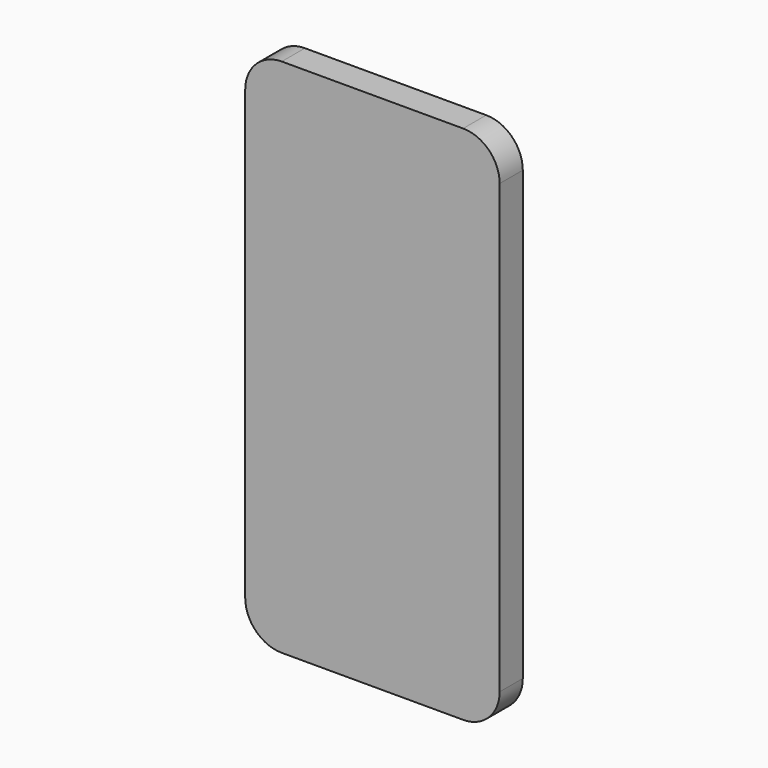
from build123d import *

# Parameters (mm, degrees)
F0_W         = 69.6
F0_H         = 142.4
F1_DEPTH     = 7.9
F2_R         = 10
F3_TEXT_SIZE = 14.5033047895
F4_DEPTH     = 0.5


# Not quite as in the source:
# - Text() gives the source's letters only with a copy of the font that has no kerning and outlines rounded to 1/6400 em; it was checked with that copy


with BuildPart() as f1:
    # F0 (on Front) → F1 (new body)
    with BuildSketch(Plane.XZ):
        Rectangle(F0_W, F0_H)
    extrude(amount=F1_DEPTH)

    # F2
    f2_edges = [f1.edges().sort_by_distance(p)[0] for p in [
        (-34.8, -3.95, 71.2),
        (34.8, -3.95, 71.2),
        (-34.8, -3.95, -71.2),
        (34.8, -3.95, -71.2),
    ]]
    fillet(f2_edges, radius=F2_R)

    # F3 (on face) → F4 (join)
    with BuildSketch(Plane(origin=(0, 0, 0), x_dir=(-1, 0, 0), z_dir=(0, 1, 0))):
        with Locations((-34.8, -10.4423794484)):
            Text('Galaxy S7', F3_TEXT_SIZE, font='Open Sans', font_style=FontStyle.BOLD, text_align=(TextAlign.LEFT, TextAlign.BOTTOM))
    extrude(amount=F4_DEPTH)


solid = f1.part
